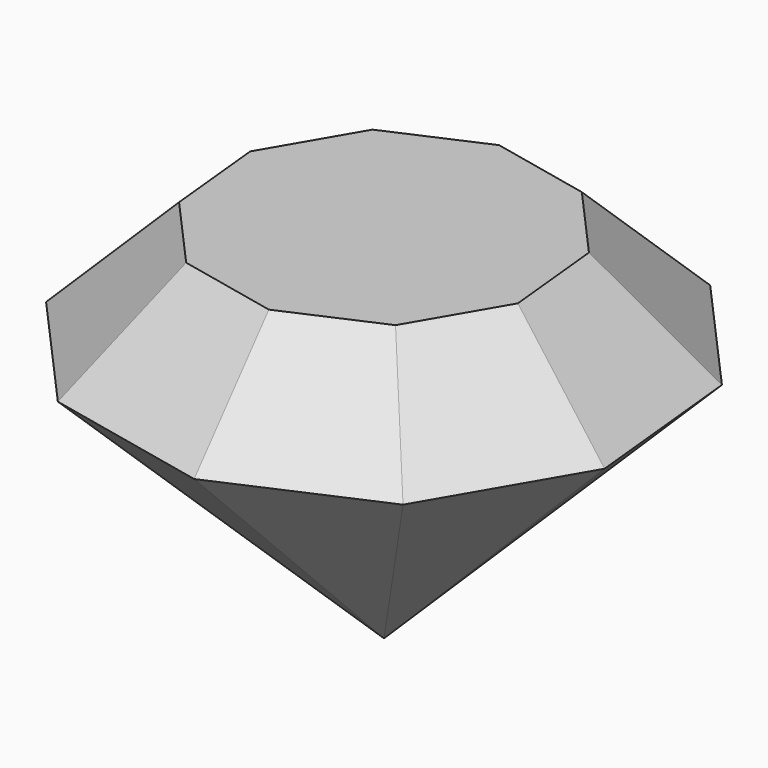
from build123d import *

# Parameters (mm, degrees)
F1_DEPTH     = 40.64
F2_SIZE      = 12.7
F3_T1_DEPTH  = 176.0479365306
F3_T3_DEPTH  = 176.0479365306
F3_T5_DEPTH  = 176.0479365306
F3_T7_DEPTH  = 176.0479365306
F3_T9_DEPTH  = 176.0479365306
F3_T11_DEPTH = 176.0479365306
F3_T13_DEPTH = 176.0479365306
F3_T15_DEPTH = 176.0479365306
F3_T17_DEPTH = 176.0479365306
F3_T19_DEPTH = 176.0479365306


# Not quite as in the source:
# - a fillet or chamfer that OpenCascade refuses, or shapes differently, is made with other operations: its cross-section is extruded or revolved along the edge and cut away or added


with BuildPart() as f1:
    # F0 (on Top) → F1 (new body)
    with BuildSketch(Plane.XY):
        Polygon((29.2412366164, 12.8835857291), (16.083875671, 27.6106074452), (-3.2169791099, 31.7913155674), (-21.2890572119, 23.8288216898), (-31.2294390474, 6.7645278386), (-29.2412366164, -12.8835857291), (-16.083875671, -27.6106074452), (3.2169791099, -31.7913155674), (21.2890572119, -23.8288216898), (31.2294390474, -6.7645278386), align=None)
    extrude(amount=F1_DEPTH)

    # F2
    f2_edges = [f1.edges().sort_by_distance(p)[0] for p in [
        (12.253018, -27.810069, 40.64),
        (26.259248, -15.296675, 40.64),
        (30.235338, 3.059529, 40.64),
        (22.662556, 20.247097, 40.64),
        (6.433448, 29.700962, 40.64),
        (-12.253018, 27.810069, 40.64),
        (-26.259248, 15.296675, 40.64),
        (-30.235338, -3.059529, 40.64),
        (-22.662556, -20.247097, 40.64),
        (-6.433448, -29.700962, 40.64),
    ]]
    chamfer(f2_edges, length=F2_SIZE)

    # F3: chamfer of 30.38856 on 10 edges, made by hand

    # F3_s2 → F3_t1 (cut)
    with BuildSketch(Plane(origin=(-86.0289159586, 18.6345004803, 0), x_dir=(0, 0, 1), z_dir=(0.9773351242, -0.2116980278, 0))):
        Polygon((0, 0.001181216), (30.38856, 30.389741216), (0, 30.389741216), align=None)
    extrude(amount=F3_T1_DEPTH, mode=Mode.SUBTRACT)

    # F3_s4 → F3_t3 (cut)
    with BuildSketch(Plane(origin=(8.8619339292, -87.5767384424, 0), x_dir=(0, 0, 1), z_dir=(-0.1006763738, 0.9949192268, 0))):
        Polygon((30.38856, 30.389741216), (0, 0.001181216), (0, 30.389741216), align=None)
    extrude(amount=F3_T3_DEPTH, mode=Mode.SUBTRACT)

    # F3_s6 → F3_t5 (cut)
    with BuildSketch(Plane(origin=(58.645770452, -65.6421556414, 0), x_dir=(0, 0, 1), z_dir=(-0.666247746, 0.7457304747, 0))):
        Polygon((0, 0.001181216), (30.38856, 30.389741216), (0, 30.389741216), align=None)
    extrude(amount=F3_T5_DEPTH, mode=Mode.SUBTRACT)

    # F3_s8 → F3_t7 (cut)
    with BuildSketch(Plane(origin=(86.0289159586, -18.6345004803, 0), x_dir=(0, 0, 1), z_dir=(-0.9773351242, 0.2116980278, 0))):
        Polygon((0, 0.001181216), (30.38856, 30.389741216), (0, 30.389741216), align=None)
    extrude(amount=F3_T7_DEPTH, mode=Mode.SUBTRACT)

    # F3_s10 → F3_t9 (cut)
    with BuildSketch(Plane(origin=(80.5519395843, 35.490900501, 0), x_dir=(0, 0, 1), z_dir=(-0.9151137034, -0.4031958704, 0))):
        Polygon((0, 0.001181216), (30.38856, 30.389741216), (0, 30.389741216), align=None)
    extrude(amount=F3_T9_DEPTH, mode=Mode.SUBTRACT)

    # F3_s12 → F3_t11 (cut)
    with BuildSketch(Plane(origin=(44.3068601486, 76.0599837822, 0), x_dir=(0, 0, 1), z_dir=(-0.5033499514, -0.8640826502, 0))):
        Polygon((0, 0.001181216), (30.38856, 30.389741216), (0, 30.389741216), align=None)
    extrude(amount=F3_T11_DEPTH, mode=Mode.SUBTRACT)

    # F3_s14 → F3_t13 (cut)
    with BuildSketch(Plane(origin=(-8.8619339292, 87.5767384424, 0), x_dir=(0, 0, 1), z_dir=(0.1006763738, -0.9949192268, 0))):
        Polygon((0, 0.001181216), (30.38856, 30.389741216), (0, 30.389741216), align=None)
    extrude(amount=F3_T13_DEPTH, mode=Mode.SUBTRACT)

    # F3_s16 → F3_t15 (cut)
    with BuildSketch(Plane(origin=(-58.645770452, 65.6421556414, 0), x_dir=(0, 0, 1), z_dir=(0.666247746, -0.7457304747, 0))):
        Polygon((0, 0.001181216), (30.38856, 30.389741216), (0, 30.389741216), align=None)
    extrude(amount=F3_T15_DEPTH, mode=Mode.SUBTRACT)

    # F3_s18 → F3_t17 (cut)
    with BuildSketch(Plane(origin=(-80.5519395843, -35.490900501, 0), x_dir=(0, 0, 1), z_dir=(0.9151137034, 0.4031958704, 0))):
        Polygon((0, 0.001181216), (30.38856, 30.389741216), (0, 30.389741216), align=None)
    extrude(amount=F3_T17_DEPTH, mode=Mode.SUBTRACT)

    # F3_s20 → F3_t19 (cut)
    with BuildSketch(Plane(origin=(-44.3068601486, -76.0599837822, 0), x_dir=(0, 0, 1), z_dir=(0.5033499514, 0.8640826502, 0))):
        Polygon((30.38856, 30.389741216), (0, 0.001181216), (0, 30.389741216), align=None)
    extrude(amount=F3_T19_DEPTH, mode=Mode.SUBTRACT)


solid = f1.part
